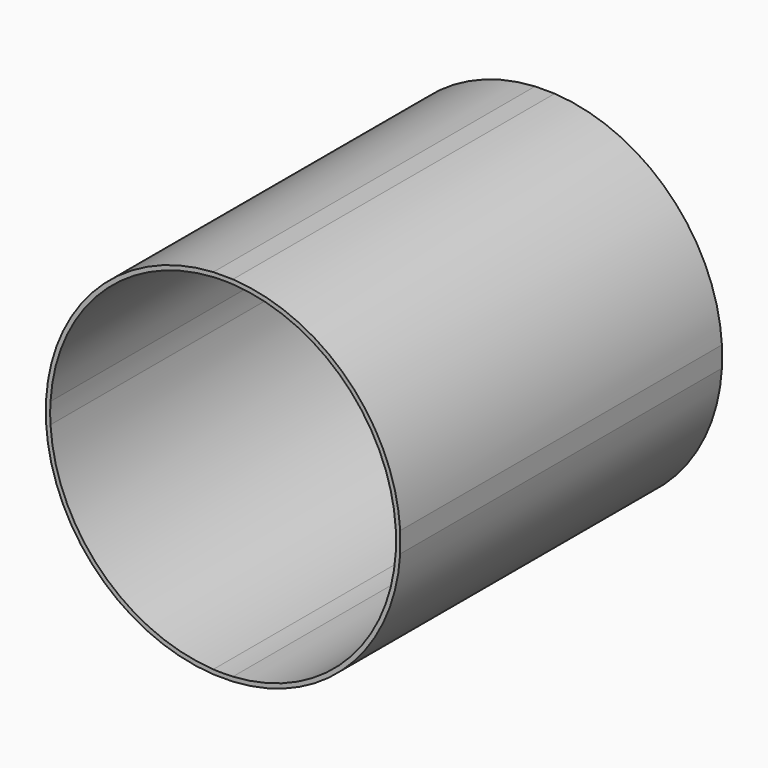
from build123d import *

# Parameters (mm, degrees)
F1_DEPTH = 25.4


# Not quite as in the source:
# - the program builds the solid bodies; features that only make, move or delete a surface that nothing else refers to are left out


with BuildPart() as f1:
    # F0 (on Front) → F1 (new body)
    with BuildSketch(Plane.XZ):
        with BuildLine():
            ThreePointArc((-11.1825731718, -0.6491680963), (-7.9102714826, -7.9308869007), (-0.6200603199, -11.1842249244))
            Line((-0.6200603199, -11.1842249244), (-0.6200603199, -10.9043848611))
            ThreePointArc((-0.6200603199, -10.9043848611), (-7.7127048151, -7.7333219534), (-10.902690713, -0.6491680963))
            Line((-10.902690713, -0.6491680963), (-11.1825731718, -0.6491680963))
        make_face()
        with BuildLine():
            Line((-10.902690713, 0.6491680963), (-11.1825731718, 0.6491680963))
            Line((-11.1825731718, 0.6491680963), (-11.1825731718, -0.6491680963))
            Line((-11.1825731718, -0.6491680963), (-10.902690713, -0.6491680963))
            ThreePointArc((-10.902690713, -0.6491680963), (-10.922, 0), (-10.902690713, 0.6491680963))
        make_face()
        with BuildLine():
            Line((-0.6200603199, 10.9043848611), (-0.6200603199, 11.1842249244))
            ThreePointArc((-0.6200603199, 11.1842249244), (-7.9102714826, 7.9308869007), (-11.1825731718, 0.6491680963))
            Line((-11.1825731718, 0.6491680963), (-10.902690713, 0.6491680963))
            ThreePointArc((-10.902690713, 0.6491680963), (-7.7127048151, 7.7333219534), (-0.6200603199, 10.9043848611))
        make_face()
        with BuildLine():
            Line((0.6200603199, 10.9043848611), (0.6200603199, 11.1842249244))
            Line((0.6200603199, 11.1842249244), (-0.6200603199, 11.1842249244))
            Line((-0.6200603199, 11.1842249244), (-0.6200603199, 10.9043848611))
            ThreePointArc((-0.6200603199, 10.9043848611), (0, 10.922), (0.6200603199, 10.9043848611))
        make_face()
        with BuildLine():
            Line((10.902690713, 0.6491680963), (11.1825731718, 0.6491680963))
            ThreePointArc((11.1825731718, 0.6491680963), (7.9102714826, 7.9308869007), (0.6200603199, 11.1842249244))
            Line((0.6200603199, 11.1842249244), (0.6200603199, 10.9043848611))
            ThreePointArc((0.6200603199, 10.9043848611), (7.7127048151, 7.7333219534), (10.902690713, 0.6491680963))
        make_face()
        with BuildLine():
            Line((11.1825731718, -0.6491680963), (11.1825731718, 0.6491680963))
            Line((11.1825731718, 0.6491680963), (10.902690713, 0.6491680963))
            ThreePointArc((10.902690713, 0.6491680963), (10.917171611, 0.3247276035), (10.922, 0))
            ThreePointArc((10.922, 0), (10.917171611, -0.3247276035), (10.902690713, -0.6491680963))
            Line((10.902690713, -0.6491680963), (11.1825731718, -0.6491680963))
        make_face()
        with BuildLine():
            ThreePointArc((0.6200603199, -11.1842249244), (7.9102714826, -7.9308869007), (11.1825731718, -0.6491680963))
            Line((11.1825731718, -0.6491680963), (10.902690713, -0.6491680963))
            ThreePointArc((10.902690713, -0.6491680963), (7.7127048151, -7.7333219534), (0.6200603199, -10.9043848611))
            Line((0.6200603199, -10.9043848611), (0.6200603199, -11.1842249244))
        make_face()
        with BuildLine():
            Line((-0.6200603199, -11.1842249244), (0.6200603199, -11.1842249244))
            Line((0.6200603199, -11.1842249244), (0.6200603199, -10.9043848611))
            ThreePointArc((0.6200603199, -10.9043848611), (0, -10.922), (-0.6200603199, -10.9043848611))
            Line((-0.6200603199, -10.9043848611), (-0.6200603199, -11.1842249244))
        make_face()
    extrude(amount=F1_DEPTH)


solid = f1.part
